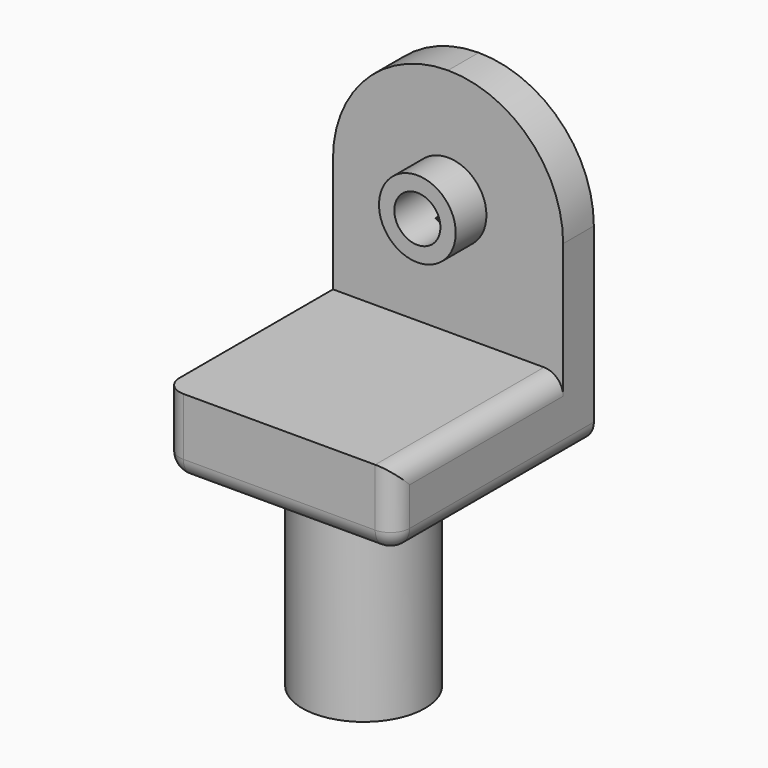
from build123d import *

# Parameters (mm, degrees)
F0_R      = 16
F1_DEPTH  = 50
F3_DEPTH  = 20
F4_W      = 60
F4_H      = 10
F5_DEPTH  = 20
F6_W      = 60
F6_H      = 10
F7_DEPTH  = 60
F8_R      = 29.99999
F9_R      = 10
F10_DEPTH = 10
F11_R     = 6
F12_DEPTH = 20.001
F14_R     = 5
F15_DEPTH = 25


# Not quite as in the source:
# - a fillet or chamfer is up to 0.001 mm smaller than in the source, because OpenCascade refuses the exact size


with BuildPart() as f1:
    # F0 (on Top) → F1 (new body)
    with BuildSketch(Plane.XY):
        with Locations((-36.3172069192, -31.1424750835)):
            Circle(F0_R)
    extrude(amount=F1_DEPTH)

    # F2 (on face) → F3 (join)
    with BuildSketch(Plane.XY.offset(50)):
        Polygon((-66.3172069192, -3.6424750835), (-66.3172069192, -31.1424750835), (-66.3172069192, -58.6424750835), (-36.3172069192, -58.6424750835), (-6.3172069192, -58.6424750835), (-6.3172069192, -31.1424750835), (-6.3172069192, -3.6424750835), (-36.3172069192, -3.6424750835), align=None)
    extrude(amount=F3_DEPTH)

    # F4 (on face) → F5 (join)
    with BuildSketch(Plane.XY.offset(70)):
        with Locations((-36.3172069192, 1.3575249165)):
            Rectangle(F4_W, F4_H)
    extrude(amount=-F5_DEPTH)

    # F6 (on face) → F7 (join)
    with BuildSketch(Plane.XY.offset(70)):
        with Locations((-36.3172069192, 1.3575249165)):
            Rectangle(F6_W, F6_H)
    extrude(amount=F7_DEPTH)

    # F8 (radius 30 in the source; OpenCascade refuses exactly that, so slightly less here)
    f8_edges = [f1.edges().sort_by_distance(p)[0] for p in [
        (-66.317207, 1.357525, 130),
        (-6.317207, 1.357525, 130),
    ]]
    fillet(f8_edges, radius=F8_R)

    # F9 (on face) → F10 (join)
    with BuildSketch(Plane.XZ.offset(3.6424750835)):
        with Locations((-36.3172069192, 100)):
            Circle(F9_R)
    extrude(amount=F10_DEPTH)

    # F11 (on face) → F12 (cut, through all)
    with BuildSketch(Plane.XZ.offset(13.6424750835)):
        with Locations((-36.3172069192, 100)):
            Circle(F11_R)
    extrude(amount=-F12_DEPTH, mode=Mode.SUBTRACT)

    # F14
    f14_edges = [f1.edges().sort_by_distance(p)[0] for p in [
        (-66.317207, -58.642475, 60),
        (-66.317207, -26.142475, 50),
        (-36.317207, -58.642475, 50),
        (-6.317207, -26.142475, 50),
        (-6.317207, -58.642475, 60),
        (-6.317207, -31.142475, 70),
    ]]
    fillet(f14_edges, radius=F14_R)

    # F6 (on face) → F15 (join)
    with BuildSketch(Plane.XY.offset(70)):
        with Locations((-36.3172069192, 1.3575249165)):
            Rectangle(F6_W, F6_H)
    extrude(amount=F15_DEPTH)


solid = f1.part
